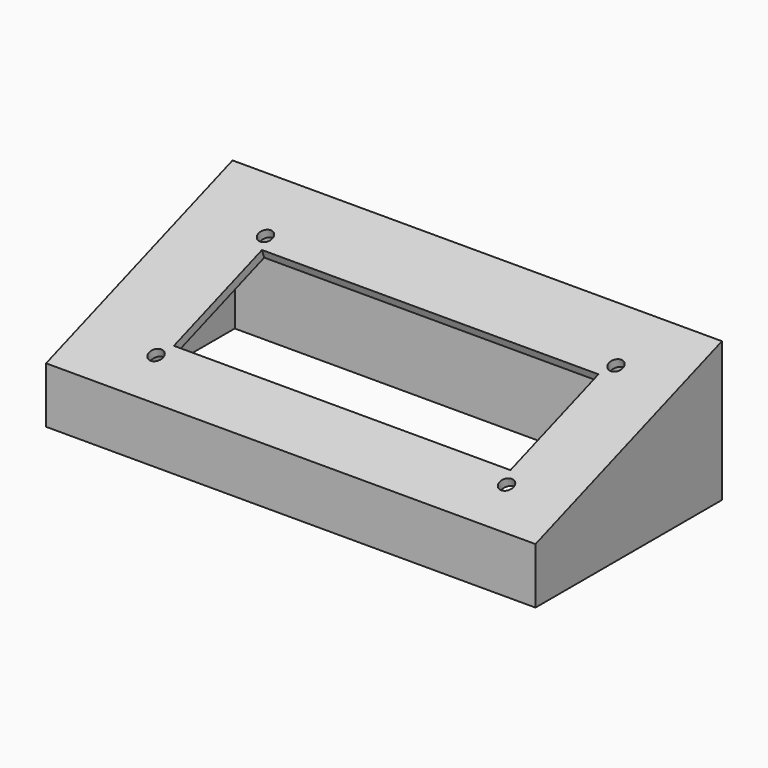
from build123d import *

# Parameters (mm, degrees)
F0_W     = 100.2
F0_H     = 45.2
F1_DEPTH = 30
F3_DEPTH = 105.001
F6_DEPTH = 105
F4_W     = 72.2
F4_H     = 25.1
F4_R     = 1.5
F7_DEPTH = 5
F8_DEPTH = 5


with BuildPart() as f1:
    # F0 (on Top) → F1 (new body)
    with BuildSketch(Plane.XY):
        Polygon((52.5, 25), (-52.5, 25), (-52.5, 4), (-52.5, -4), (-52.5, -25), (52.5, -25), (52.5, -4), (52.5, 4), align=None)
        Rectangle(F0_W, F0_H, mode=Mode.SUBTRACT)
    extrude(amount=F1_DEPTH)

    # F2 (on face) → F3 (cut, through all)
    with BuildSketch(Plane.YZ.offset(52.5)):
        Polygon((-25, 12), (25, 30), (-25, 30), align=None)
    extrude(amount=-F3_DEPTH, mode=Mode.SUBTRACT)

    # F5 (on face) → F6 (join)
    with BuildSketch(Plane(origin=(-52.5, 0, 0), x_dir=(0, -1, 0), z_dir=(-1, 0, 0))):
        Polygon((25, 12), (-25, 30), (-25, 28.0869124432), (25, 10.0869124432), align=None)
    extrude(amount=-F6_DEPTH)

    # F4 (on face) → F7 (cut)
    with BuildSketch(Plane(origin=(0, -6.6926345609, 18.5906515581), x_dir=(1, 0, 0), z_dir=(0, -0.3387194683, 0.9408874119))):
        with Locations((1.5, 5.7432311296)):
            Rectangle(F4_W, F4_H)
        with Locations((39.1, -9.9067688704)):
            Circle(F4_R)
        with Locations((39.1, 21.2932311296)):
            Circle(F4_R)
        with Locations((-36.1, -9.9067688704)):
            Circle(F4_R)
        with Locations((-36.1, 21.2932311296)):
            Circle(F4_R)
    extrude(amount=-F7_DEPTH, mode=Mode.SUBTRACT)

    # F5 (on face) → F8 (cut)
    with BuildSketch(Plane(origin=(-52.5, 0, 0), x_dir=(0, -1, 0), z_dir=(-1, 0, 0))):
        Polygon((-3.4536782682, 11.6150599721), (-17.5669894462, 16.6958519962), (-18.9218673193, 12.9323023487), (-4.8085561413, 7.8515103246), align=None)
    extrude(amount=-F8_DEPTH, mode=Mode.SUBTRACT)


solid = f1.part
